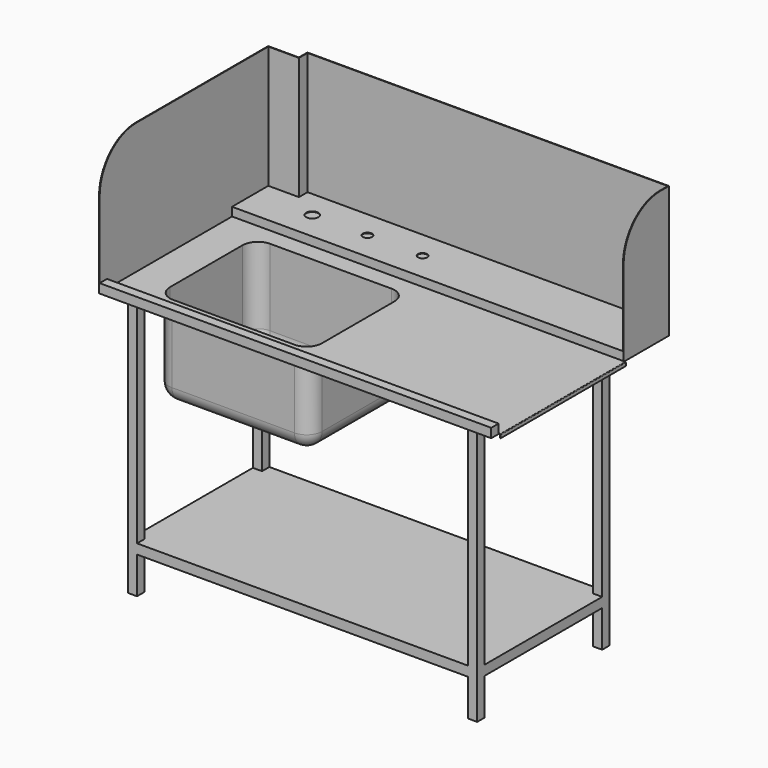
from build123d import *

# Parameters (mm, degrees)
F1_DEPTH    = 30
F2_W        = 1278
F2_H        = 510
F3_DEPTH    = 28
F4_W        = 500
F4_H        = 400
F5_DEPTH    = 300
F6_T        = 2
F6_T3_DEPTH = 34
F6_T5_DEPTH = 404
F6_T7_DEPTH = 504
F6_T9_DEPTH = 32
F7_R        = 50
F8_R        = 25
F9_DEPTH    = 2
F10_R       = 15
F10_R_2     = 20
F11_DEPTH   = 30
F12_W       = 510
F12_H       = 2
F13_DEPTH   = 5
F14_W       = 510
F14_H       = 2
F15_ANGLE   = 90
F16_W       = 2
F16_H       = 510
F17_DEPTH   = 10
F19_DEPTH   = 400
F20_R       = 150
F21_W       = 30
F21_H       = 30
F22_DEPTH   = 850
F23_W       = 30
F23_H       = 30
F24_DEPTH   = 1080
F25_W       = 30
F25_H       = 30
F26_DEPTH   = 480
F28_DEPTH   = 2


# Not quite as in the source:
# - a shell that OpenCascade refuses in one call is made with other operations: the cavity is built on its own and cut out


with BuildPart() as f1:
    # F0 (on Top) → F1 (new body)
    with BuildSketch(Plane.XY):
        Polygon((0, 690), (0, 0), (1280, 0), (1280, 725), (100, 725), (100, 690), align=None)
    extrude(amount=F1_DEPTH)

    # F2 (on face) → F3 (cut)
    with BuildSketch(Plane.XY.offset(30)):
        with Locations((641, 285)):
            Rectangle(F2_W, F2_H)
    extrude(amount=-F3_DEPTH, mode=Mode.SUBTRACT)

    # F4 (on face) → F5 (join)
    with BuildSketch(Plane(origin=(0, 0, 0), x_dir=(1, 0, 0), z_dir=(0, 0, -1))):
        with Locations((370, -285)):
            Rectangle(F4_W, F4_H)
    extrude(amount=F5_DEPTH)

    # F6: shell of thickness 2, made by hand


with BuildPart() as f6_core1:
    # F6_t2: copy of F1
    add(f1.part)

    # the walls: a layer under each face that stays
    f6_faces = [f6_core1.faces().sort_by_distance(p)[0] for p in [
        (0, 345, 15),
        (50, 690, 15),
        (640, 0, 15),
        (640, 362.5, 0),
        (213.3333333333, 604.1666666667, 30),
        (100, 707.5, 15),
        (1280, 604.1666666667, 25),
        (690, 725, 15),
        (620, 285, -150),
        (370, 485, -150),
        (120, 285, -150),
        (370, 85, -150),
        (641, 540, 16),
        (2, 285, 16),
        (641, 30, 16),
        (370, 285, -300),
    ]]
    thicken(f6_faces, amount=-F6_T, mode=Mode.SUBTRACT)

    # F6_s4 → F6_t3 (cut)
    with BuildSketch(Plane.XY.offset(-2)):
        Polygon((99.98, 690.02), (100, 688), (102, 688), (102, 690), align=None)
    extrude(amount=F6_T3_DEPTH, mode=Mode.SUBTRACT)

    # F6_s6 → F6_t5 (cut)
    with BuildSketch(Plane.XZ.offset(-487)):
        Polygon((620.02, -0.02), (620, 2), (618, 2), (618, 0), align=None)
        Polygon((119.98, -0.02), (120, 2), (122, 2), (122, 0), align=None)
    extrude(amount=F6_T5_DEPTH, mode=Mode.SUBTRACT)

    # F6_s8 → F6_t7 (cut)
    with BuildSketch(Plane.YZ.offset(118)):
        Polygon((485.02, -0.02), (485, 2), (483, 2), (483, 0), align=None)
        Polygon((84.98, -0.02), (85, 2), (87, 2), (87, 0), align=None)
    extrude(amount=F6_T7_DEPTH, mode=Mode.SUBTRACT)

    # F6_s10 → F6_t9 (cut)
    with BuildSketch(Plane.XY):
        Polygon((2.02, 539.98), (2, 542), (0, 542), (0, 540), align=None)
        Polygon((2.02, 30.02), (0, 30), (0, 28), (2, 28), align=None)
    extrude(amount=F6_T9_DEPTH, mode=Mode.SUBTRACT)


with BuildPart() as f1_1:
    add(f1.part)

    # what is left inside the walls is the cavity
    f6_cavity = [f6_core1.part.solids().sort_by_distance(p)[0] for p in [
        (640, 10.666667, 2.02),
        (640, 602.333333, 27.98),
        (370, 351, -297.98),
    ]]
    add(f6_cavity, mode=Mode.SUBTRACT)

    # F7
    f7_edges = [f1_1.edges().sort_by_distance(p)[0] for p in [
        (122, 483, -148),
        (618, 483, -148),
        (122, 87, -148),
        (618, 87, -148),
        (618, 285, -298),
        (370, 483, -298),
        (122, 285, -298),
        (370, 87, -298),
        (120, 85, -150),
        (370, 85, -300),
        (620, 85, -150),
        (620, 285, -300),
        (620, 485, -150),
        (370, 485, -300),
        (120, 485, -150),
        (120, 285, -300),
    ]]
    fillet(f7_edges, radius=F7_R)

    # F8 (on face) → F9 (cut, through all)
    with BuildSketch(Plane.XY.offset(-298)):
        with Locations((488, 353)):
            Circle(F8_R)
    extrude(amount=-F9_DEPTH, mode=Mode.SUBTRACT)

    # F10 (on face) → F11 (cut, through all)
    with BuildSketch(Plane.XY.offset(30)):
        with Locations((550, 632.5)):
            Circle(F10_R)
        with Locations((370, 632.5)):
            Circle(F10_R)
        with Locations((190, 632.5)):
            Circle(F10_R_2)
    extrude(amount=-F11_DEPTH, mode=Mode.SUBTRACT)

    # F12 (on face) → F13 (join)
    with BuildSketch(Plane.YZ.offset(1280)):
        with Locations((285, 1)):
            Rectangle(F12_W, F12_H)
    extrude(amount=F13_DEPTH)

    # F14 (on face) → F15 (revolve)
    with BuildSketch(Plane.YZ.offset(1285)):
        with Locations((285, 1)):
            Rectangle(F14_W, F14_H)
    revolve(axis=Axis((1285, 285, 0), (0, 1, 0)), revolution_arc=F15_ANGLE)

    # F16 (on face) → F17 (join)
    with BuildSketch(Plane(origin=(0, 0, 0), x_dir=(1, 0, 0), z_dir=(0, 0, -1))):
        with Locations((1286, -285)):
            Rectangle(F16_W, F16_H)
    extrude(amount=F17_DEPTH)

    # F18 (on face) → F19 (join)
    with BuildSketch(Plane.XY.offset(30)):
        Polygon((1278, 540), (1280, 540), (1280, 725), (100, 725), (100, 690), (0, 690), (0, 0), (2, 0), (2, 688), (102, 688), (102, 723), (1278, 723), align=None)
    extrude(amount=F19_DEPTH)

    # F20
    f20_edges = [f1_1.edges().sort_by_distance(p)[0] for p in [
        (1279, 540, 430),
        (1, 0, 430),
    ]]
    fillet(f20_edges, radius=F20_R)

    # F21 (on face) → F22 (join)
    with BuildSketch(Plane(origin=(0, 0, 0), x_dir=(1, 0, 0), z_dir=(0, 0, -1))):
        with Locations((85, -45)):
            Rectangle(F21_W, F21_H)
        with Locations((1195, -45)):
            Rectangle(F21_W, F21_H)
        with Locations((1195, -555)):
            Rectangle(F21_W, F21_H)
        with Locations((85, -555)):
            Rectangle(F21_W, F21_H)
    extrude(amount=F22_DEPTH)

    # F23 (on face) → F24 (join, through all)
    with BuildSketch(Plane.YZ.offset(100)):
        with Locations((45, -715)):
            Rectangle(F23_W, F23_H)
        with Locations((555, -715)):
            Rectangle(F23_W, F23_H)
    extrude(amount=F24_DEPTH)

    # F25 (on face) → F26 (join, through all)
    with BuildSketch(Plane(origin=(0, 60, 0), x_dir=(-1, 0, 0), z_dir=(0, 1, 0))):
        with Locations((-1195, -715)):
            Rectangle(F25_W, F25_H)
        with Locations((-85, -715)):
            Rectangle(F25_W, F25_H)
    extrude(amount=F26_DEPTH)

    # F27 (on face) → F28 (join)
    with BuildSketch(Plane.XY.offset(-700)):
        Polygon((100, 60), (100, 30), (1180, 30), (1180, 60), (1210, 60), (1210, 540), (1180, 540), (1180, 570), (100, 570), (100, 540), (70, 540), (70, 60), align=None)
    extrude(amount=F28_DEPTH)


solid = f1_1.part
